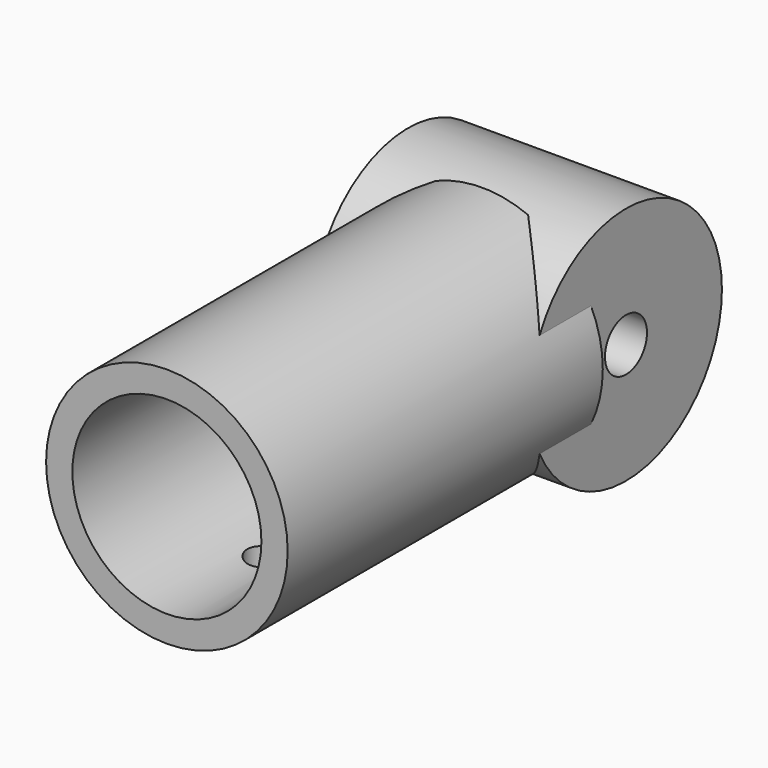
from build123d import *

# Parameters (mm, degrees)
F2_R     = 13.7
F2_R_2   = 3
F3_DEPTH = 12.45
F1_R     = 13.8
F1_R_2   = 10.8
F4_DEPTH = 45
F6_D     = 4
F6_DEPTH = 13.8010001


with BuildPart() as f3:
    # F2 (on Right) → F3 (new body, symmetric)
    with BuildSketch(Plane.YZ):
        Circle(F2_R)
        Circle(F2_R_2, mode=Mode.SUBTRACT)
    extrude(amount=F3_DEPTH, both=True)

    # F1 (on offset) → F4 (join)
    with BuildSketch(Plane.XZ.offset(50)):
        Circle(F1_R)
        Circle(F1_R_2, mode=Mode.SUBTRACT)
    extrude(amount=-F4_DEPTH)

    # F6 (through all, one way)
    with BuildSketch(Plane.XY):
        with Locations((0, -36)):
            Circle(F6_D / 2)
    extrude(amount=-F6_DEPTH, mode=Mode.SUBTRACT)


solid = f3.part
